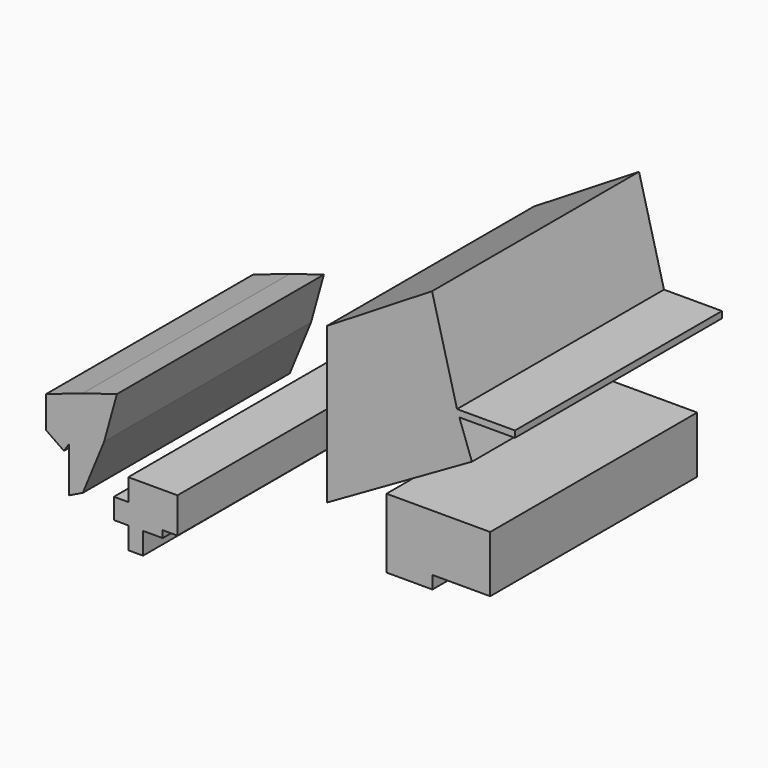
from build123d import *

# Parameters (mm, degrees)
F1_DEPTH = 254
F3_DEPTH = 254
F2_W     = 56.7163527012
F2_H     = 29.4544659555
F2_H_2   = 26.1025242507
F2_W_2   = 45.0822561979
F2_H_3   = 12.60291785
F2_W_3   = 14.0579044819
F2_H_4   = 20.1796069741
F2_W_4   = 14.5426690578
F2_H_5   = 21.498978138
F2_H_6   = 21.4939191937
F2_W_5   = 19.3063616753
F2_H_7   = 13.3150070906
F2_H_8   = 6.8645998836


with BuildPart() as f1:
    # F0 (on Front) → F1 (new body)
    with BuildSketch(Plane.XZ):
        Polygon((-195.0813531876, -10.2526498958), (-231.1204969883, -22.5838702172), (-208.6613327265, -58.4072656929), (-196.0759667594, -13.7795502332), align=None)
        Polygon((-208.6613327265, -58.4072656929), (-231.1204969883, -22.5838702172), (-231.1204969883, -53.8410842419), (-213.5470360518, -65.9608095884), align=None)
        Polygon((-196.0759667594, -13.7795502332), (-208.6613327265, -58.4072656929), (-174.1891205311, -45.3221611679), align=None)
        Polygon((-174.1891205311, -45.3221611679), (-208.6613327265, -58.4072656929), (-195.0813531876, -96.2715595961), align=None)
        Polygon((-195.0813531876, -96.2715595961), (-208.6613327265, -58.4072656929), (-208.6613327265, -102.8021946549), align=None)
        Polygon((-161.59465909, 0), (-195.0813531876, -10.2526498958), (-196.0759667594, -13.7795502332), (-174.1891205311, -45.3221611679), align=None)
    extrude(amount=F1_DEPTH)


with BuildPart() as f3:
    # F2 (on Front) → F3 (new body)
    with BuildSketch(Plane.XZ):
        Polygon((147.7846652269, 189.5339041948), (44.4636456668, 125.8510947227), (172.3015010357, 95.6252366304), align=None)
        Polygon((172.3015010357, 95.6252366304), (44.4636456668, 125.8510947227), (44.4636456668, -26.7503317446), align=None)
        Polygon((172.3015010357, 89.2322733998), (172.3015010357, 95.6252366304), (44.4636456668, -26.7503317446), (186.8948787451, 54.8904277384), (174.5918008958, 89.2322733998), align=None)
        Polygon((229.1480302811, 95.6252366304), (172.3015010357, 95.6252366304), (174.5918008958, 89.2322733998), (229.1480302811, 89.2322733998), align=None)
        Polygon((174.5918008958, 89.2322733998), (172.3015010357, 95.6252366304), (172.3015010357, 89.2322733998), align=None)
    extrude(amount=F3_DEPTH)


with BuildPart() as f3b:
    # F2 (on Front) → F3, piece 2 (new body)
    with BuildSketch(Plane.XZ):
        with Locations((176.5156239271, -14.7272329777)):
            Rectangle(F2_W, F2_H)
        Polygon((148.1574475765, -29.4544659555), (148.1574475765, 0), (114.2245531082, 0), (103.0751913786, 0), (103.0751913786, -29.4544659555), align=None)
        with Locations((176.5156239271, -42.5057280809)):
            Rectangle(F2_W, F2_H_2)
        with Locations((125.6163194776, -42.5057280809)):
            Rectangle(F2_W_2, F2_H_2)
        with Locations((125.6163194776, -61.8584491313)):
            Rectangle(F2_W_2, F2_H_3)
    extrude(amount=F3_DEPTH)


with BuildPart() as f3c:
    # F2 (on Front) → F3, piece 3 (new body)
    with BuildSketch(Plane.XZ):
        with Locations((-157.4808359146, -99.7486896813)):
            Rectangle(F2_W_3, F2_H_4)
        Polygon((-135.9092146158, -89.6588861942), (-150.4518836737, -89.6588861942), (-150.4518836737, -109.8384931684), (-135.9092146158, -109.8384931684), (-135.9092146158, -102.9738932848), align=None)
        with Locations((-143.1805491447, -78.9093971252)):
            Rectangle(F2_W_4, F2_H_5)
        with Locations((-143.1805491447, -120.5854527652)):
            Rectangle(F2_W_4, F2_H_6)
        Polygon((-135.9092146158, -68.1599080563), (-135.9092146158, -89.6588861942), (-116.6028529406, -89.6588861942), (-116.6028529406, -102.9738932848), (-102.1160781384, -102.9738932848), (-102.1160781384, -68.1599080563), align=None)
        with Locations((-126.2560337782, -96.3163897395)):
            Rectangle(F2_W_5, F2_H_7)
        with Locations((-126.2560337782, -106.4061932266)):
            Rectangle(F2_W_5, F2_H_8)
    extrude(amount=F3_DEPTH)


solid = Compound([f1.part, f3.part, f3b.part, f3c.part])
